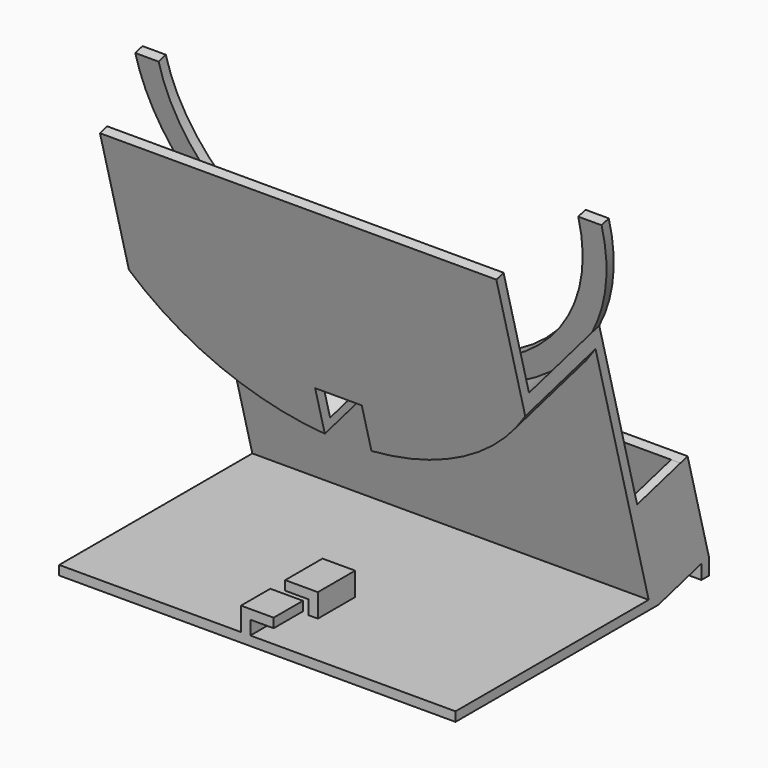
from build123d import *

# Parameters (mm, degrees)
F1_DEPTH  = 85
F3_DEPTH  = 2
F5_DEPTH  = 2
F7_DEPTH  = 25
F9_DEPTH  = 17.5
F11_DEPTH = 2
F13_DEPTH = 10
F15_DEPTH = 2
F16_W     = 7
F16_H     = 10
F17_DEPTH = 5
F18_W     = 5
F18_H     = 3
F19_DEPTH = 25
F20_W     = 7
F20_H     = 7.8445977569
F21_DEPTH = 5
F22_W     = 5
F22_H     = 3
F23_DEPTH = 8


with BuildPart() as f1:
    # F0 (on Right) → F1 (new body)
    with BuildSketch(Plane.YZ):
        Polygon((-54.3862693012, 2), (-54.3862693012, 0), (0, 0), (11.522961568, 3.0875682466), (11.522961568, 0), (13.522961568, 0), (13.522961568, 3.6234666314), (13.0053234778, 5.555318284), (7.8289425758, 24.8738348098), (5.8970909232, 24.3561967196), (11.0734718253, 5.0376801938), (-0.5176380902, 1.9318516526), (-23.2389682748, 86.7290103171), (-25.1708199274, 86.2113722269), (-2.6064507457, 2), align=None)
    extrude(amount=F1_DEPTH)

    # F2 (on face) → F3 (join)
    with BuildSketch(Plane.YZ.offset(85)):
        Polygon((11.0734718253, 5.0376801938), (5.8970909232, 24.3561967196), (-5.6940189923, 21.2503681784), (-0.5176380902, 1.9318516526), align=None)
    extrude(amount=-F3_DEPTH)

    # F4 (on face) → F5 (join)
    with BuildSketch(Plane(origin=(0, 0, 0), x_dir=(0, -1, 0), z_dir=(-1, 0, 0))):
        Polygon((5.6940189923, 21.2503681784), (-5.8970909232, 24.3561967196), (-11.0734718253, 5.0376801938), (0.5176380902, 1.9318516526), align=None)
    extrude(amount=-F5_DEPTH)

    # F6 (on face) → F7 (cut)
    with BuildSketch(Plane(origin=(0, -1.9318516526, -0.5176380902), x_dir=(1, 0, 0), z_dir=(0, -0.9659258263, -0.2588190451))):
        with BuildLine():
            ThreePointArc((0, 61.2673163635), (56.1930639376, 39.5179905915), (92.5, 87.6064507457))
            ThreePointArc((92.5, 87.6064507457), (28.8069360624, 135.6949108999), (0, 61.2673163635))
        make_face()
    extrude(amount=-F7_DEPTH, mode=Mode.SUBTRACT)

    # F8 (on face) → F9 (join)
    with BuildSketch(Plane(origin=(0, -1.9318516526, -0.5176380902), x_dir=(1, 0, 0), z_dir=(0, -0.9659258263, -0.2588190451))):
        with BuildLine():
            ThreePointArc((85, 61.2673163636), (42.5, 37.6064507457), (0, 61.2673163636))
            Line((0, 61.2673163636), (0, 57.6439742125))
            ThreePointArc((0, 57.6439742125), (42.5, 35.6064507457), (85, 57.6439742125))
            Line((85, 57.6439742125), (85, 61.2673163636))
        make_face()
    extrude(amount=F9_DEPTH)

    # F10 (on face) → F11 (join)
    with BuildSketch(Plane(origin=(0, -18.8355536126, -5.0469713795), x_dir=(1, 0, 0), z_dir=(0, -0.9659258263, -0.2588190451))):
        with BuildLine():
            Line((0, 61.2673163636), (0, 57.6439742125))
            ThreePointArc((0, 57.6439742125), (42.5, 35.6064507457), (85, 57.6439742125))
            Line((85, 57.6439742125), (85, 61.2673163636))
            Line((85, 61.2673163636), (85, 87.6064507457))
            Line((85, 87.6064507457), (0, 87.6064507457))
            Line((0, 87.6064507457), (0, 61.2673163636))
        make_face()
    extrude(amount=F11_DEPTH)

    # F12 (on face) → F13 (cut)
    with BuildSketch(Plane(origin=(0, -20.7674052652, -5.5646094697), x_dir=(1, 0, 0), z_dir=(0, -0.9659258263, -0.2588190451))):
        with BuildLine():
            Line((37.5, 45.8473935673), (37.5, 35.8473935673))
            ThreePointArc((37.5, 35.8473935673), (42.5, 35.6064507457), (47.5, 35.8473935673))
            Line((47.5, 35.8473935673), (47.5, 45.8473935673))
            Line((47.5, 45.8473935673), (37.5, 45.8473935673))
        make_face()
    extrude(amount=-F13_DEPTH, mode=Mode.SUBTRACT)

    # F14 (on face) → F15 (join)
    with BuildSketch(Plane(origin=(0, 0, 0), x_dir=(-1, 0, 0), z_dir=(0, 0.9659258263, 0.2588190451))):
        with BuildLine():
            ThreePointArc((-92.5, 87.6064507457), (-42.5, 37.6064507457), (7.5, 87.6064507457))
            Line((7.5, 87.6064507457), (2.5, 87.6064507457))
            ThreePointArc((2.5, 87.6064507457), (-42.5, 42.6064507457), (-87.5, 87.6064507457))
            Line((-87.5, 87.6064507457), (-92.5, 87.6064507457))
        make_face()
    extrude(amount=-F15_DEPTH)

    # F16 (on face) → F17 (join)
    with BuildSketch(Plane.XY.offset(2)):
        with Locations((42.5, -37.5416715443)):
            Rectangle(F16_W, F16_H)
    extrude(amount=F17_DEPTH)

    # F18 (on face) → F19 (cut)
    with BuildSketch(Plane.XZ.offset(42.5416715443)):
        with Locations((41.5, 3.5)):
            Rectangle(F18_W, F18_H)
    extrude(amount=-F19_DEPTH, mode=Mode.SUBTRACT)

    # F20 (on face) → F21 (join)
    with BuildSketch(Plane.XY.offset(2)):
        with Locations((42.5, -50.4639704227)):
            Rectangle(F20_W, F20_H)
    extrude(amount=F21_DEPTH)

    # F22 (on face) → F23 (cut)
    with BuildSketch(Plane.XZ.offset(54.3862693012)):
        with Locations((43.5, 3.5)):
            Rectangle(F22_W, F22_H)
    extrude(amount=-F23_DEPTH, mode=Mode.SUBTRACT)


solid = f1.part
